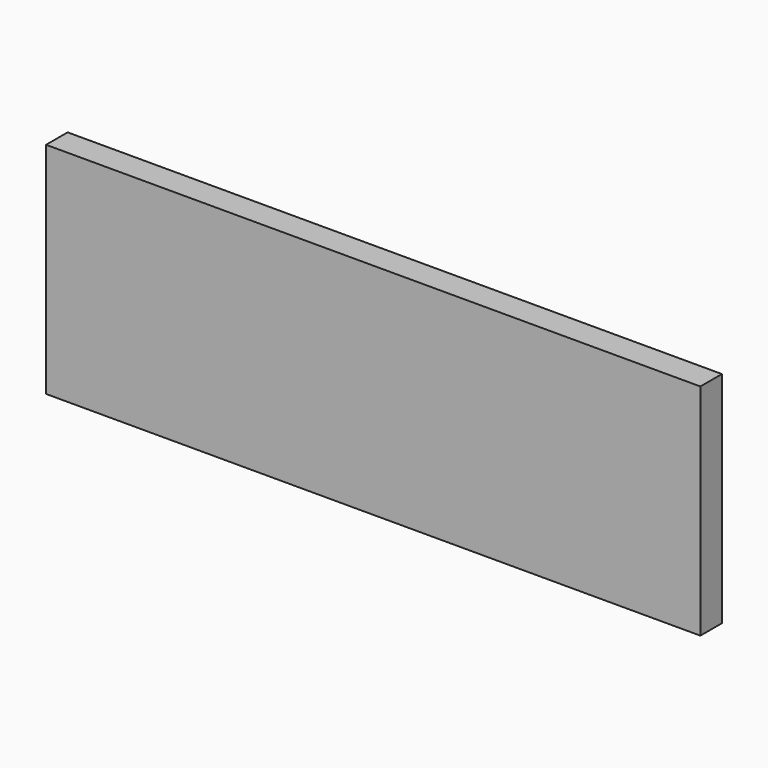
from build123d import *

# Parameters (mm, degrees)
F1_W     = 404.8252
F1_H     = 135.7376
F2_DEPTH = 16.6624
F3_R     = 6.35
F4_DEPTH = 12.7


# Not quite as in the source:
# - a variable given as a bare number and used for a length is read in inches; the dataset says mm whatever the document's units were


with BuildPart() as f2:
    # F1 (on Front) → F2 (new body)
    with BuildSketch(Plane.XZ):
        with Locations((-202.4126, 67.8688)):
            Rectangle(F1_W, F1_H)
    extrude(amount=F2_DEPTH)

    # F3 (on face) → F4 (join)
    with BuildSketch(Plane(origin=(0, 0, 0), x_dir=(-1, 0, 0), z_dir=(0, 1, 0))):
        with Locations((202.4126, 67.8688)):
            Circle(F3_R)
    extrude(amount=F4_DEPTH)


solid = f2.part
